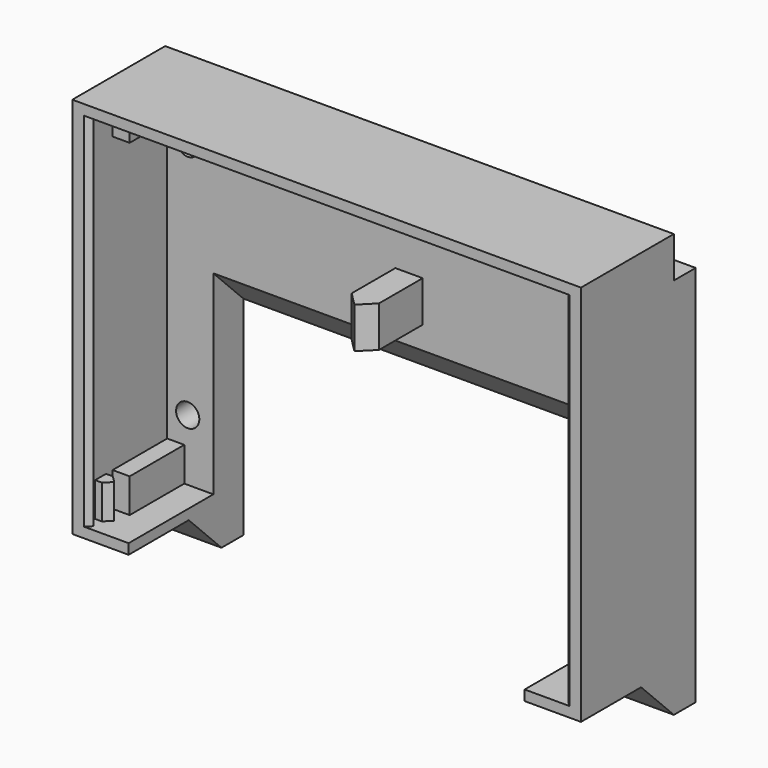
from build123d import *

# Parameters (mm, degrees)
F0_W         = 74.5
F0_H         = 56
F1_DEPTH     = 17
F2_T         = -1.5
F3_W         = 2.5
F3_H         = 5
F4_DEPTH     = 10
F5_W         = 1.6
F5_H         = 53
F7_DEPTH     = 1.2
F6_W         = 1.6
F6_H         = 53
F8_DEPTH     = 1.2
F9_W         = 0.5
F9_H         = 1.6
F9_W_2       = 5.5
F10_DEPTH    = 1.2
F11_SIZE     = 0.8
F12_SIZE2    = 0.79999
F12_SIZE     = 0.79999
F13_W        = 2
F13_H        = 5
F14_DEPTH    = 2
F15_W        = 2
F15_H        = 5
F16_DEPTH    = 2
F17_T1_DEPTH = 7.571682988
F17_T3_DEPTH = 53
F18_W        = 75.0788375735
F18_H        = 56
F19_DEPTH    = 4
F20_W        = 58
F20_H        = 30
F20_R        = 1.7
F21_DEPTH    = 25
F22_T1_DEPTH = 8.25
F22_T3_DEPTH = 8.25
F22_T5_DEPTH = 58
F23_W        = 4
F23_H        = 6
F24_DEPTH    = 10
F25_SIZE     = 1.99999


# Not quite as in the source:
# - a fillet or chamfer that OpenCascade refuses, or shapes differently, is made with other operations: its cross-section is extruded or revolved along the edge and cut away or added
# - a fillet or chamfer is up to 0.001 mm smaller than in the source, because OpenCascade refuses the exact size


with BuildPart() as f1:
    # F0 (on Front) → F1 (new body)
    with BuildSketch(Plane.XZ):
        with Locations((-37.25, 28)):
            Rectangle(F0_W, F0_H)
    extrude(amount=F1_DEPTH)

    # F2
    f2_openings = [f1.faces().sort_by_distance(p)[0] for p in [
        (-37.25, -17, 28),
    ]]
    offset(amount=F2_T, openings=f2_openings)

    # F3 (on face) → F4 (join)
    with BuildSketch(Plane.XZ.offset(1.5)):
        with Locations((-71.75, 52)):
            Rectangle(F3_W, F3_H)
        with Locations((-2.75, 52)):
            Rectangle(F3_W, F3_H)
        with Locations((-2.75, 4)):
            Rectangle(F3_W, F3_H)
        with Locations((-71.75, 4)):
            Rectangle(F3_W, F3_H)
    extrude(amount=F4_DEPTH)

    # F5 (on face) → F7 (join)
    with BuildSketch(Plane.YZ.offset(-73)):
        with Locations((-16.2, 28)):
            Rectangle(F5_W, F5_H)
    extrude(amount=F7_DEPTH)

    # F6 (on face) → F8 (join)
    with BuildSketch(Plane(origin=(-1.5, 0, 0), x_dir=(0, -1, 0), z_dir=(-1, 0, 0))):
        with Locations((16.2, 28)):
            Rectangle(F6_W, F6_H)
    extrude(amount=F8_DEPTH)

    # F9 (on face) → F10 (join)
    with BuildSketch(Plane(origin=(0, 0, 54.5), x_dir=(1, 0, 0), z_dir=(0, 0, -1))):
        with Locations((-73.25, 13.5)):
            Rectangle(F9_W, F9_H)
        with Locations((-70.25, 13.5)):
            Rectangle(F9_W_2, F9_H)
        with Locations((-4.25, 13.5)):
            Rectangle(F9_W_2, F9_H)
    extrude(amount=F10_DEPTH)

    # F11
    f11_edges = [f1.edges().sort_by_distance(p)[0] for p in [
        (-4.25, -14.3, 53.3),
        (-70.25, -14.3, 53.3),
    ]]
    chamfer(f11_edges, length=F11_SIZE)

    # F12 (size 0.8 and 0.8 in the source; OpenCascade refuses exactly that, so slightly less here)
    f12_edges = [f1.edges().sort_by_distance(p)[0] for p in [
        (-70.25, -12.7, 53.3),
        (-4.25, -12.7, 53.3),
    ]]
    chamfer(f12_edges, length=F12_SIZE, length2=F12_SIZE2)

    # F13 (on face) → F14 (join)
    with BuildSketch(Plane(origin=(-1.5, 0, 0), x_dir=(0, -1, 0), z_dir=(-1, 0, 0))):
        with Locations((13.7, 4)):
            Rectangle(F13_W, F13_H)
    extrude(amount=F14_DEPTH)

    # F15 (on face) → F16 (join)
    with BuildSketch(Plane.YZ.offset(-73)):
        with Locations((-13.7, 4)):
            Rectangle(F15_W, F15_H)
    extrude(amount=F16_DEPTH)

    # F17: chamfer of 1 on 8 edges, made by hand

    # F17_s2 → F17_t1 (cut)
    with BuildSketch(Plane.XY.offset(1.5)):
        Polygon((-72, -14.7), (-71, -13.7), (-71, -14.7), align=None)
        Polygon((-72, -12.7), (-71, -13.7), (-71, -12.7), align=None)
        Polygon((-3.5, -13.7), (-2.5, -14.7), (-3.5, -14.7), align=None)
        Polygon((-2.5, -12.7), (-3.5, -13.7), (-3.5, -12.7), align=None)
    extrude(amount=F17_T1_DEPTH, mode=Mode.SUBTRACT)

    # F17_s4 → F17_t3 (cut)
    with BuildSketch(Plane.XY.offset(1.5)):
        Polygon((-1.7, -17), (-2.7, -16), (-2.7, -17), align=None)
        Polygon((-2.7, -16.4), (-1.7, -15.4), (-2.7, -15.4), align=None)
        Polygon((-71.8, -16), (-72.8, -17), (-71.8, -17), align=None)
        Polygon((-72.8, -15.4), (-71.8, -16.4), (-71.8, -15.4), align=None)
    extrude(amount=F17_T3_DEPTH, mode=Mode.SUBTRACT)

    # F18 (on face) → F19 (join)
    with BuildSketch(Plane(origin=(0, 0, 0), x_dir=(-1, 0, 0), z_dir=(0, 1, 0))):
        with Locations((37.5394187868, 22)):
            Rectangle(F18_W, F18_H)
    extrude(amount=F19_DEPTH)

    # F20 (on face) → F21 (cut)
    with BuildSketch(Plane(origin=(0, 4, 0), x_dir=(-1, 0, 0), z_dir=(0, 1, 0))):
        with Locations((37.25, 9)):
            Rectangle(F20_W, F20_H)
        with Locations((4.5017562807, 10.5)):
            Circle(F20_R)
        with Locations((4.5017562807, 45.5)):
            Circle(F20_R)
        with Locations((69.9982437193, 10.5)):
            Circle(F20_R)
        with Locations((69.9982437193, 45.5)):
            Circle(F20_R)
    extrude(amount=-F21_DEPTH, mode=Mode.SUBTRACT)

    # F22: chamfer of 6 on 3 edges, made by hand

    # F22_s2 → F22_t1 (join)
    with BuildSketch(Plane.YZ.offset(-74.5)):
        Polygon((-6, 0), (0, -6), (0, 0), align=None)
    extrude(amount=F22_T1_DEPTH)

    # F22_s4 → F22_t3 (join)
    with BuildSketch(Plane.YZ.offset(-8.25)):
        Polygon((-6, 0), (0, -6), (0, 0), align=None)
    extrude(amount=F22_T3_DEPTH)

    # F22_s6 → F22_t5 (cut)
    with BuildSketch(Plane.YZ.offset(-66.25)):
        Polygon((4.5, 24), (-1.5, 30), (-1.5, 24), align=None)
    extrude(amount=F22_T5_DEPTH, mode=Mode.SUBTRACT)

    # F23 (on face) → F24 (join)
    with BuildSketch(Plane.XZ.offset(1.5)):
        with Locations((-37.5844355226, 36.3401113749)):
            Rectangle(F23_W, F23_H)
    extrude(amount=F24_DEPTH)

    # F25 (size 2 in the source; OpenCascade refuses exactly that, so slightly less here)
    f25_edges = [f1.edges().sort_by_distance(p)[0] for p in [
        (-39.584436, -11.5, 36.340111),
        (-35.584436, -11.5, 36.340111),
    ]]
    chamfer(f25_edges, length=F25_SIZE)


solid = f1.part
